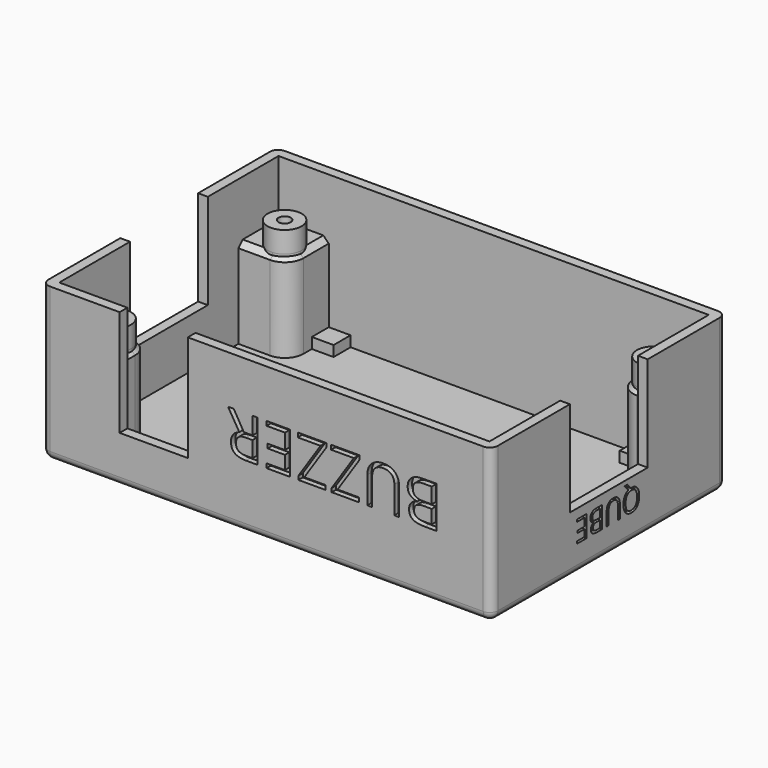
from build123d import *

# Parameters (mm, degrees)
F0_W          = 82.5
F0_H          = 53.85
F0_W_2        = 78.94
F0_H_2        = 50.29
F1_DEPTH      = 28.15
F2_W          = 82.5
F2_H          = 1.55
F3_DEPTH      = 53.85
F4_R          = 3.125
F4_R_2        = 1.125
F5_DEPTH      = 21.9
F7_DEPTH      = 18
F8_R          = 1.5
F9_T3_DEPTH   = 5.8401010127
F9_S4_R       = 3.125
F9_T5_DEPTH   = 5
F9_T8_DEPTH   = 5.8401010127
F9_S9_R       = 3.125
F9_T10_DEPTH  = 5
F9_T13_DEPTH  = 5.8401010127
F9_S14_R      = 3.125
F9_T15_DEPTH  = 5
F9_T18_DEPTH  = 5.8401010127
F9_S19_R      = 3.125
F9_T20_DEPTH  = 5
F9_T23_DEPTH  = 5.8401010127
F9_S24_R      = 3.125
F9_T25_DEPTH  = 5
F9_T28_DEPTH  = 5.8401010127
F9_S29_R      = 3.125
F9_T30_DEPTH  = 5
F9_T33_DEPTH  = 5.8401010127
F9_S34_R      = 3.125
F9_T35_DEPTH  = 5
F9_T38_DEPTH  = 5.8401010127
F9_S39_R      = 3.125
F9_T40_DEPTH  = 5
F9_T43_ANGLE  = 90
F9_S44_R      = 3.125
F9_T45_DEPTH  = 4
F9_T48_ANGLE  = 90
F9_S49_R      = 3.125
F9_T50_DEPTH  = 4
F9_T53_ANGLE  = 90
F9_S54_R      = 3.125
F9_T55_DEPTH  = 4
F9_T58_ANGLE  = 90
F9_S59_R      = 3.125
F9_T60_DEPTH  = 4
F10_DEPTH     = 7
F11_W         = 17.85
F11_H         = 17.5
F12_DEPTH     = 137.9
F13_W         = 12.5
F13_H         = 19.5
F14_DEPTH     = 25
F15_TEXT_SIZE = 10.0787401575
F16_DEPTH     = 0.85
F18_TEXT_SIZE = 5.5035833333
F19_DEPTH     = 0.85
F17_TEXT_SIZE = 5.5035773253
F20_DEPTH     = 0.85
F21_W         = 4.175
F21_H         = 2
F22_DEPTH     = 15
F23_W         = 4.175
F23_H         = 2
F24_DEPTH     = 15
F25_TEXT_SIZE = 10.6965278068
F26_DEPTH     = 1


# Not quite as in the source:
# - a fillet or chamfer that OpenCascade refuses, or shapes differently, is made with other operations: its cross-section is extruded or revolved along the edge and cut away or added
# - Text() gives the source's letters only with a copy of the font that has no kerning and outlines rounded to 1/6400 em; it was checked with that copy


with BuildPart() as f1:
    # F0 (on Top) → F1 (new body)
    with BuildSketch(Plane.XY):
        with Locations((41.25, 26.925)):
            Rectangle(F0_W, F0_H)
        with Locations((41.25, 26.925)):
            Rectangle(F0_W_2, F0_H_2, mode=Mode.SUBTRACT)
    extrude(amount=F1_DEPTH)

    # F2 (on Front) → F3 (join)
    with BuildSketch(Plane.XZ):
        with Locations((41.25, 0.775)):
            Rectangle(F2_W, F2_H)
    extrude(amount=-F3_DEPTH)

    # F4 (on Top) → F5 (join)
    with BuildSketch(Plane.XY):
        with Locations((7.36, 46.4899988616)):
            Circle(F4_R)
        with Locations((7.36, 46.4899988616)):
            Circle(F4_R_2, mode=Mode.SUBTRACT)
        with Locations((7.36, 7.36)):
            Circle(F4_R)
        with Locations((7.36, 7.36)):
            Circle(F4_R_2, mode=Mode.SUBTRACT)
        with Locations((75.1400032783, 7.36)):
            Circle(F4_R)
        with Locations((75.1400032783, 7.36)):
            Circle(F4_R_2, mode=Mode.SUBTRACT)
        with Locations((75.1400032783, 46.4899986982)):
            Circle(F4_R)
        with Locations((75.1400032783, 46.4899986982)):
            Circle(F4_R_2, mode=Mode.SUBTRACT)
    extrude(amount=F5_DEPTH)

    # F6 (on Top) → F7 (join)
    with BuildSketch(Plane.XY):
        with BuildLine():
            Line((0, 11), (0, 0))
            Line((0, 0), (11, 0))
            Line((11, 0), (11, 7.6201010127))
            ThreePointArc((11, 7.6201010127), (10.0100505063, 10.0100505063), (7.6201010127, 11))
            Line((7.6201010127, 11), (0, 11))
        make_face()
        with BuildLine():
            Line((0, 53.85), (0, 42.85))
            Line((0, 42.85), (7.6201010127, 42.85))
            ThreePointArc((7.6201010127, 42.85), (10.0100505063, 43.8399494937), (11, 46.2298989873))
            Line((11, 46.2298989873), (11, 53.85))
            Line((11, 53.85), (0, 53.85))
        make_face()
        with BuildLine():
            Line((71.5, 7.6201010127), (71.5, 0))
            Line((71.5, 0), (82.5, 0))
            Line((82.5, 0), (82.5, 11))
            Line((82.5, 11), (74.8798989873, 11))
            ThreePointArc((74.8798989873, 11), (72.4899494937, 10.0100505063), (71.5, 7.6201010127))
        make_face()
        with BuildLine():
            Line((74.8798989873, 42.85), (82.5, 42.85))
            Line((82.5, 42.85), (82.5, 53.85))
            Line((82.5, 53.85), (71.5, 53.85))
            Line((71.5, 53.85), (71.5, 46.2298989873))
            ThreePointArc((71.5, 46.2298989873), (72.4899494937, 43.8399494937), (74.8798989873, 42.85))
        make_face()
    extrude(amount=F7_DEPTH)

    # F8
    f8_edges = [f1.edges().sort_by_distance(p)[0] for p in [
        (41.25, 53.85, 0),
        (0, 26.925, 0),
        (41.25, 0, 0),
        (82.5, 26.925, 0),
        (82.5, 53.85, 14.075),
        (82.5, 0, 14.075),
        (0, 0, 14.075),
        (0, 53.85, 14.075),
    ]]
    fillet(f8_edges, radius=F8_R)

    # F9: chamfer of 1 on 12 edges, made by hand


with BuildPart() as f9_tool1:
    # F9_s2 → F9_t3 (new body)
    with BuildSketch(Plane.XZ.offset(-46.2298989873)):
        Polygon((10, 18), (11, 17), (11, 18), align=None)
    extrude(amount=-F9_T3_DEPTH)

    # F9_s4 → F9_t5 (cut, symmetric)
    with BuildSketch(Plane.XY.offset(17.5)):
        with Locations((7.36, 46.4899988616)):
            Circle(F9_S4_R)
    extrude(amount=F9_T5_DEPTH, both=True, mode=Mode.SUBTRACT)


with BuildPart() as f9_tool6:
    # F9_s7 → F9_t8 (new body)
    with BuildSketch(Plane.YZ.offset(1.78)):
        Polygon((42.85, 17), (43.85, 18), (42.85, 18), align=None)
    extrude(amount=F9_T8_DEPTH)

    # F9_s9 → F9_t10 (cut, symmetric)
    with BuildSketch(Plane.XY.offset(17.5)):
        with Locations((7.36, 46.4899988616)):
            Circle(F9_S9_R)
    extrude(amount=F9_T10_DEPTH, both=True, mode=Mode.SUBTRACT)


with BuildPart() as f9_tool11:
    # F9_s12 → F9_t13 (new body)
    with BuildSketch(Plane.YZ.offset(7.6201010127)):
        Polygon((10, 18), (11, 17), (11, 18), align=None)
    extrude(amount=-F9_T13_DEPTH)

    # F9_s14 → F9_t15 (cut, symmetric)
    with BuildSketch(Plane.XY.offset(17.5)):
        with Locations((7.36, 7.36)):
            Circle(F9_S14_R)
    extrude(amount=F9_T15_DEPTH, both=True, mode=Mode.SUBTRACT)


with BuildPart() as f9_tool16:
    # F9_s17 → F9_t18 (new body)
    with BuildSketch(Plane.XZ.offset(-1.78)):
        Polygon((11, 17), (10, 18), (11, 18), align=None)
    extrude(amount=-F9_T18_DEPTH)

    # F9_s19 → F9_t20 (cut, symmetric)
    with BuildSketch(Plane.XY.offset(17.5)):
        with Locations((7.36, 7.36)):
            Circle(F9_S19_R)
    extrude(amount=F9_T20_DEPTH, both=True, mode=Mode.SUBTRACT)


with BuildPart() as f9_tool21:
    # F9_s22 → F9_t23 (new body)
    with BuildSketch(Plane.XZ.offset(-7.6201010127)):
        Polygon((72.5, 18), (71.5, 17), (71.5, 18), align=None)
    extrude(amount=F9_T23_DEPTH)

    # F9_s24 → F9_t25 (cut, symmetric)
    with BuildSketch(Plane.XY.offset(17.5)):
        with Locations((75.1400032783, 7.36)):
            Circle(F9_S24_R)
    extrude(amount=F9_T25_DEPTH, both=True, mode=Mode.SUBTRACT)


with BuildPart() as f9_tool26:
    # F9_s27 → F9_t28 (new body)
    with BuildSketch(Plane.YZ.offset(80.72)):
        Polygon((10, 18), (11, 17), (11, 18), align=None)
    extrude(amount=-F9_T28_DEPTH)

    # F9_s29 → F9_t30 (cut, symmetric)
    with BuildSketch(Plane.XY.offset(17.5)):
        with Locations((75.1400032783, 7.36)):
            Circle(F9_S29_R)
    extrude(amount=F9_T30_DEPTH, both=True, mode=Mode.SUBTRACT)


with BuildPart() as f9_tool31:
    # F9_s32 → F9_t33 (new body)
    with BuildSketch(Plane.XZ.offset(-52.07)):
        Polygon((71.5, 17), (72.5, 18), (71.5, 18), align=None)
    extrude(amount=F9_T33_DEPTH)

    # F9_s34 → F9_t35 (cut, symmetric)
    with BuildSketch(Plane.XY.offset(17.5)):
        with Locations((75.1400032783, 46.4899986982)):
            Circle(F9_S34_R)
    extrude(amount=F9_T35_DEPTH, both=True, mode=Mode.SUBTRACT)


with BuildPart() as f9_tool36:
    # F9_s37 → F9_t38 (new body)
    with BuildSketch(Plane.YZ.offset(74.8798989873)):
        Polygon((43.85, 18), (42.85, 17), (42.85, 18), align=None)
    extrude(amount=F9_T38_DEPTH)

    # F9_s39 → F9_t40 (cut, symmetric)
    with BuildSketch(Plane.XY.offset(17.5)):
        with Locations((75.1400032783, 46.4899986982)):
            Circle(F9_S39_R)
    extrude(amount=F9_T40_DEPTH, both=True, mode=Mode.SUBTRACT)


with BuildPart() as f9_tool41:
    # F9_s42 → F9_t43 (revolve)
    with BuildSketch(Plane.XZ.offset(-7.6201010127)):
        Polygon((10, 18), (11, 17), (11, 18), align=None)
    revolve(axis=Axis((7.6201010127, 7.6201010127, 18), (0, 0, 1)), revolution_arc=F9_T43_ANGLE)

    # F9_s44 → F9_t45 (cut, symmetric)
    with BuildSketch(Plane.XY.offset(17.5)):
        with Locations((7.36, 7.36)):
            Circle(F9_S44_R)
    extrude(amount=F9_T45_DEPTH, both=True, mode=Mode.SUBTRACT)


with BuildPart() as f9_tool46:
    # F9_s47 → F9_t48 (revolve)
    with BuildSketch(Plane.YZ.offset(7.6201010127)):
        Polygon((43.85, 18), (42.85, 17), (42.85, 18), align=None)
    revolve(axis=Axis((7.6201010127, 46.2298989873, 18), (0, 0, 1)), revolution_arc=F9_T48_ANGLE)

    # F9_s49 → F9_t50 (cut, symmetric)
    with BuildSketch(Plane.XY.offset(17.5)):
        with Locations((7.36, 46.4899988616)):
            Circle(F9_S49_R)
    extrude(amount=F9_T50_DEPTH, both=True, mode=Mode.SUBTRACT)


with BuildPart() as f9_tool51:
    # F9_s52 → F9_t53 (revolve)
    with BuildSketch(Plane.XZ.offset(-46.2298989873)):
        Polygon((72.5, 18), (71.5, 17), (71.5, 18), align=None)
    revolve(axis=Axis((74.8798989873, 46.2298989873, 18), (0, 0, 1)), revolution_arc=F9_T53_ANGLE)

    # F9_s54 → F9_t55 (cut, symmetric)
    with BuildSketch(Plane.XY.offset(17.5)):
        with Locations((75.1400032783, 46.4899986982)):
            Circle(F9_S54_R)
    extrude(amount=F9_T55_DEPTH, both=True, mode=Mode.SUBTRACT)


with BuildPart() as f9_tool56:
    # F9_s57 → F9_t58 (revolve)
    with BuildSketch(Plane.YZ.offset(74.8798989873)):
        Polygon((10, 18), (11, 17), (11, 18), align=None)
    revolve(axis=Axis((74.8798989873, 7.6201010127, 18), (0, 0, 1)), revolution_arc=F9_T58_ANGLE)

    # F9_s59 → F9_t60 (cut, symmetric)
    with BuildSketch(Plane.XY.offset(17.5)):
        with Locations((75.1400032783, 7.36)):
            Circle(F9_S59_R)
    extrude(amount=F9_T60_DEPTH, both=True, mode=Mode.SUBTRACT)


with BuildPart() as f1_1:
    add(f1.part)

    # F9_t61: cut F9_tool1, F9_tool6, F9_tool11, F9_tool16, F9_tool21, F9_tool26, F9_tool31, F9_tool36, F9_tool41, F9_tool46, F9_tool51, F9_tool56
    add([f9_tool1.part, f9_tool6.part, f9_tool11.part, f9_tool16.part, f9_tool21.part, f9_tool26.part, f9_tool31.part, f9_tool36.part, f9_tool41.part, f9_tool46.part, f9_tool51.part, f9_tool56.part], mode=Mode.SUBTRACT)

    # F10 (cut): faces of the model
    f10_faces = [f1_1.faces().sort_by_distance(p)[0] for p in [
        (7.36, 7.36, 18),
        (7.36, 46.4899988616, 18),
        (75.1400032783, 46.4899986982, 18),
        (75.1400032783, 7.36, 18),
    ]]
    extrude(f10_faces, amount=-F10_DEPTH, mode=Mode.SUBTRACT)

    # F11 (on Right) → F12 (cut)
    with BuildSketch(Plane.YZ):
        with Locations((26.925, 19.4)):
            Rectangle(F11_W, F11_H)
    extrude(amount=F12_DEPTH, mode=Mode.SUBTRACT)

    # F13 (on Front) → F14 (cut)
    with BuildSketch(Plane.XZ):
        with Locations((20.53, 18.4)):
            Rectangle(F13_W, F13_H)
    extrude(amount=-F14_DEPTH, mode=Mode.SUBTRACT)

    # F15 (on face) → F16 (cut)
    with BuildSketch(Plane(origin=(0, 53.85, 0), x_dir=(-1, 0, 0), z_dir=(0, 1, 0))):
        with Locations(Location((-6.5997692943, 18.1038358109), (0, 0, 180))):
            Text('INTCS.COM.AU', F15_TEXT_SIZE, font='Open Sans', text_align=(TextAlign.LEFT, TextAlign.BOTTOM))
    extrude(amount=-F16_DEPTH, mode=Mode.SUBTRACT)

    # F18 (on face) → F19 (cut)
    with BuildSketch(Plane.YZ.offset(82.5)):
        with Locations(Location((34.240990267, 8.8747626887), (0, 0, 180))):
            Text('QUBE', F18_TEXT_SIZE, font='Open Sans', text_align=(TextAlign.LEFT, TextAlign.BOTTOM))
    extrude(amount=-F19_DEPTH, mode=Mode.SUBTRACT)

    # F17 (on face) → F20 (cut)
    with BuildSketch(Plane(origin=(0, 0, 0), x_dir=(0, -1, 0), z_dir=(-1, 0, 0))):
        with Locations(Location((-14.8002535105, 7.5747545177), (0, 0, -180))):
            Text('SCANNER', F17_TEXT_SIZE, font='Open Sans', text_align=(TextAlign.LEFT, TextAlign.BOTTOM))
    extrude(amount=-F20_DEPTH, mode=Mode.SUBTRACT)

    # F21 (on Right) → F22 (join)
    with BuildSketch(Plane.YZ):
        with Locations((50.2625, 2.4933788916)):
            Rectangle(F21_W, F21_H)
        with Locations((3.5875, 2.5)):
            Rectangle(F21_W, F21_H)
    extrude(amount=F22_DEPTH)

    # F23 (on face) → F24 (join)
    with BuildSketch(Plane.YZ.offset(82.5)):
        with Locations((3.5875, 2.5)):
            Rectangle(F23_W, F23_H)
        with Locations((50.2625, 2.5)):
            Rectangle(F23_W, F23_H)
    extrude(amount=-F24_DEPTH)

    # F25 (on face) → F26 (cut)
    with BuildSketch(Plane.XZ):
        with Locations(Location((73.4773361683, 19.3514988571), (0, 0, -180))):
            Text('BUZZER', F25_TEXT_SIZE, font='Open Sans', text_align=(TextAlign.LEFT, TextAlign.BOTTOM))
    extrude(amount=-F26_DEPTH, mode=Mode.SUBTRACT)


solid = f1_1.part
